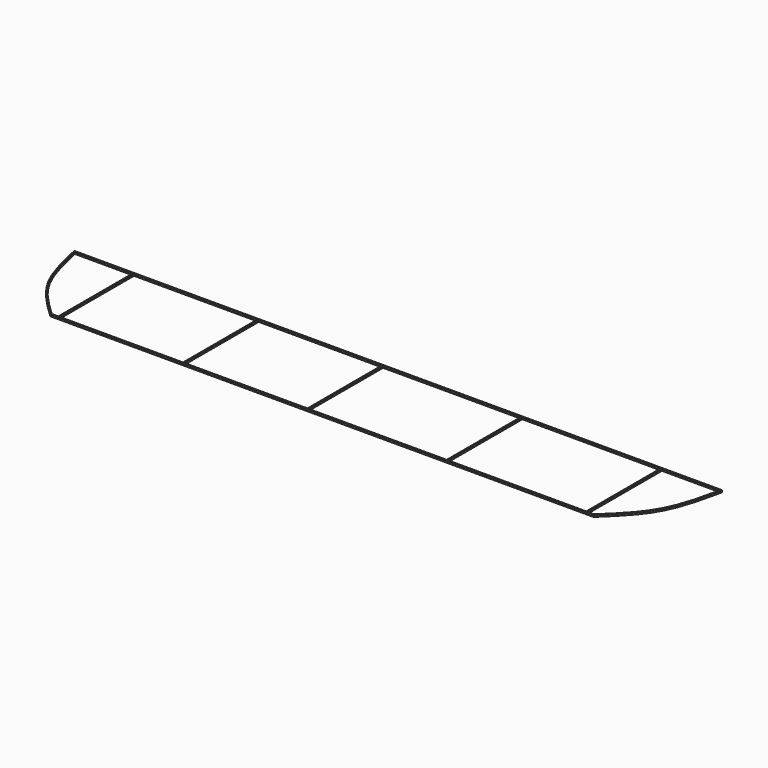
from build123d import *

# Parameters (mm, degrees)
F0_W     = 41.599999994
F0_H     = 31.349999994
F0_W_2   = 41.499999994
F0_W_3   = 46.499999994
F0_W_4   = 46.599999994
F1_DEPTH = 0.6


# Not quite as in the source:
# - the dataset's text gives a spline's control points without its knots; the knots are read off the source's solid


with BuildPart() as f1:
    # F0 (on Top) → F1 (new body)
    with BuildSketch(Plane.XY):
        with BuildLine():
            ThreePointArc((98.814183375, 2.1706994269), (98.774829603, 2.3390928353), (98.6188949823, 2.4138554825))
            Line((98.6188949823, 2.4138554825), (78.6188949823, 2.4138554825))
            Line((78.6188949823, 2.4138554825), (-99.1811050177, 2.4138554825))
            Line((-99.1811050177, 2.4138554825), (-119.1811050177, 2.4138554825))
            ThreePointArc((-119.1811050177, 2.4138554825), (-119.3370396383, 2.3390928353), (-119.3763934104, 2.1706994269))
            add(Edge.make_bspline(
                [(-119.3763934104, 2.1706994269), (-118.6750890411, -1.0028207378), (-117.6222269238, -5.7696436228), (-115.6517108062, -11.7472049252), (-113.7502708188, -15.9475927615), (-111.2731578198, -19.7507572978), (-107.3878156711, -24.3980784692), (-104.044191919, -27.5701231915), (-101.8187503844, -29.6812436391)],
                knots=[0, 0, 0, 0, 0.25, 0.375, 0.5, 0.625, 0.75, 1, 1, 1, 1], degree=3))
            ThreePointArc((-101.8187503844, -29.6812436391), (-101.7552001492, -29.7219129588), (-101.6811050177, -29.7361445235))
            Line((-101.6811050177, -29.7361445235), (-99.1811050177, -29.7361445235))
            Line((-99.1811050177, -29.7361445235), (78.6188949823, -29.7361445235))
            Line((78.6188949823, -29.7361445235), (81.1188949823, -29.7361445235))
            ThreePointArc((81.1188949823, -29.7361445235), (81.1929901139, -29.7219129588), (81.2565403491, -29.6812436391))
            add(Edge.make_bspline(
                [(98.814183375, 2.1706994269), (98.1128790058, -1.0028207378), (97.0600168885, -5.7696436228), (95.0895007709, -11.7472049252), (93.1880607835, -15.9475927615), (90.7109477845, -19.7507572978), (86.8256056358, -24.3980784692), (83.4819818837, -27.5701231915), (81.2565403491, -29.6812436391)],
                knots=[0, 0, 0, 0, 0.25, 0.375, 0.5, 0.625, 0.75, 1, 1, 1, 1], degree=3))
        make_face()
        with Locations((-78.1811050177, -13.6611445205)):
            Rectangle(F0_W, F0_H, mode=Mode.SUBTRACT)
        with BuildLine():
            Line((-118.9320790489, 2.0138554765), (-99.3811050206, 2.0138554765))
            Line((-99.3811050206, 2.0138554765), (-99.3811050206, -29.3361445175))
            Line((-99.3811050206, -29.3361445175), (-101.6013333005, -29.3361445175))
            add(Edge.make_bspline(
                [(-118.9320790489, 2.0138554765), (-118.2486155861, -1.0783210622), (-117.2089880442, -5.7463917634), (-115.277031776, -11.6048663309), (-113.3974044946, -15.7559795008), (-110.952902669, -19.5092973502), (-107.1176304003, -24.09816661), (-103.8073987294, -27.2433707019), (-101.6013333005, -29.3361445175)],
                knots=[0.0063852918, 0.0063852918, 0.0063852918, 0.0063852918, 0.25, 0.375, 0.5, 0.625, 0.75, 0.997832841, 0.997832841, 0.997832841, 0.997832841], degree=3))
        make_face(mode=Mode.SUBTRACT)
        with Locations((-36.2311050177, -13.6611445205)):
            Rectangle(F0_W_2, F0_H, mode=Mode.SUBTRACT)
        with Locations((8.1688949823, -13.6611445205)):
            Rectangle(F0_W_3, F0_H, mode=Mode.SUBTRACT)
        with Locations((55.1188949823, -13.6611445205)):
            Rectangle(F0_W_4, F0_H, mode=Mode.SUBTRACT)
        with BuildLine():
            Line((78.8188949174, 2.0138554765), (98.3698689298, 2.0138554765))
            add(Edge.make_bspline(
                [(98.3698689298, 2.0138554765), (97.6864054722, -1.0783210382), (96.6467779336, -5.7463917142), (94.7148216728, -11.6048662593), (92.8351943914, -15.7559794292), (90.3906925658, -19.5092972786), (86.5554202753, -24.0981665644), (83.245188576, -27.243370678), (81.0391231218, -29.3361445175)],
                knots=[0.0063852936, 0.0063852936, 0.0063852936, 0.0063852936, 0.25, 0.375, 0.5, 0.625, 0.75, 0.9978328438, 0.9978328438, 0.9978328438, 0.9978328438], degree=3))
            Line((81.0391231218, -29.3361445175), (78.8188949174, -29.3361445175))
            Line((78.8188949174, -29.3361445175), (78.8188949174, 2.0138554765))
        make_face(mode=Mode.SUBTRACT)
    extrude(amount=F1_DEPTH)


solid = f1.part
